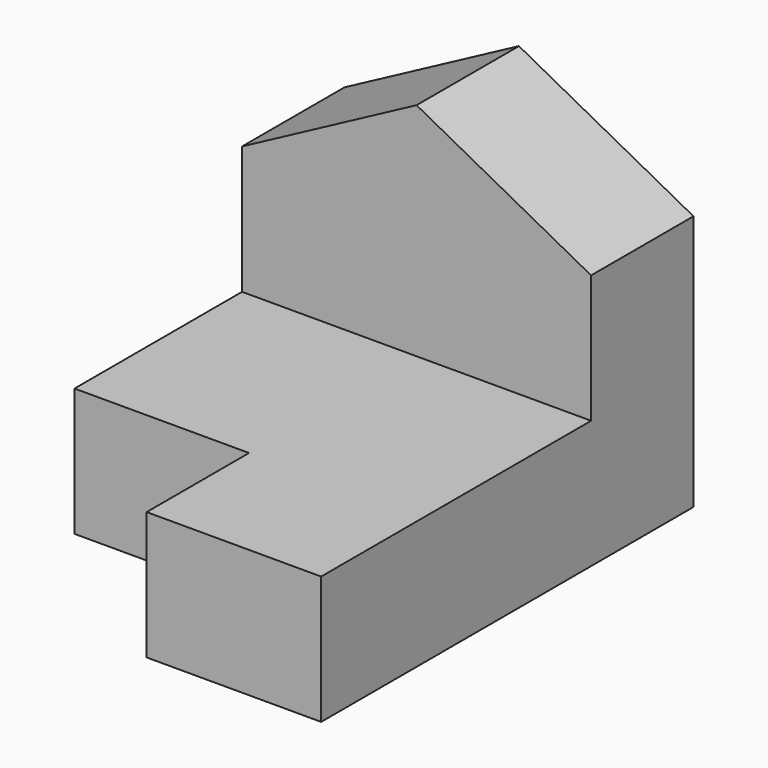
from build123d import *

# Parameters (mm, degrees)
F1_DEPTH  = 30
F2_W      = 11
F2_H      = 15
F3_DEPTH  = 11
F4_W      = 15
F4_H      = 8
F5_DEPTH  = 11
F6_ANGLE  = -90
F8_DEPTH  = 11
F10_DEPTH = 11


with BuildPart() as f1:
    # F0 (on Front) → F1 (new body)
    with BuildSketch(Plane.XZ):
        Polygon((0, 30), (0, 0), (40, 0), (40, 11), (11, 11), (11, 30), align=None)
    extrude(amount=F1_DEPTH)

    # F2 (on face) → F3 (cut, through all)
    with BuildSketch(Plane.XY.offset(11)):
        with Locations((34.5, -22.5)):
            Rectangle(F2_W, F2_H)
    extrude(amount=-F3_DEPTH, mode=Mode.SUBTRACT)

    # F4 (on face) → F5 (cut, through all)
    with BuildSketch(Plane.YZ.offset(11)):
        with Locations((-22.5, 26)):
            Rectangle(F4_W, F4_H)
    extrude(amount=-F5_DEPTH, mode=Mode.SUBTRACT)


with BuildPart() as f1_1:
    # F6: moved
    add(f1.part.rotate(Axis((0, 0, 15), (0, 0, 1)), F6_ANGLE))

    # F7 (on face) → F8 (join, through all)
    with BuildSketch(Plane.XZ.offset(11)):
        Polygon((-15, 22), (-15, 30), (-30, 22), align=None)
    extrude(amount=-F8_DEPTH)

    # F9 (on face) → F10 (cut, through all)
    with BuildSketch(Plane.XZ.offset(11)):
        Polygon((0, 30), (-15, 30), (0, 22), align=None)
    extrude(amount=-F10_DEPTH, mode=Mode.SUBTRACT)


solid = f1_1.part
